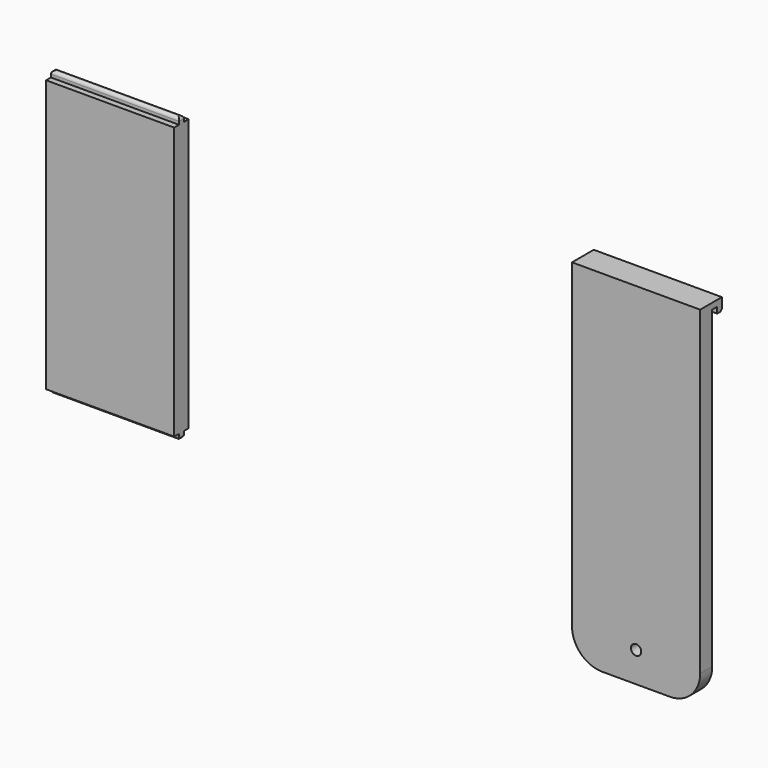
from build123d import *

# Parameters (mm, degrees)
F0_W      = 53.848
F0_H      = 114.3
F1_DEPTH  = 7.62
F2_W      = 2.54
F2_H      = 2.54
F3_DEPTH  = 53.848
F4_R      = 1.26999
F5_R      = 1.26999
F6_W      = 53.848
F6_H      = 147.32
F7_DEPTH  = 6.35
F8_R      = 12.7
F9_W      = 53.848
F9_H      = 5.08
F10_DEPTH = 5.08
F11_W     = 2.54
F11_H     = 2.54
F12_DEPTH = 76.2
F13_SIZE  = 0.762
F14_R     = 2.159
F15_DEPTH = 25.4


# Not quite as in the source:
# - a fillet or chamfer is up to 0.001 mm smaller than in the source, because OpenCascade refuses the exact size


with BuildPart() as f1:
    # F0 (on Front) → F1 (new body)
    with BuildSketch(Plane.XZ):
        with Locations((-110.2400206625, 2.555437386)):
            Rectangle(F0_W, F0_H)
    extrude(amount=F1_DEPTH)

    # F2 (on face) → F3 (join)
    with BuildSketch(Plane(origin=(-137.1640206625, 0, 0), x_dir=(0, -1, 0), z_dir=(-1, 0, 0))):
        with Locations((3.81, -55.864562614)):
            Rectangle(F2_W, F2_H)
        with Locations((3.81, 60.975437386)):
            Rectangle(F2_W, F2_H)
    extrude(amount=-F3_DEPTH)

    # F4 (radius 1.27 in the source; OpenCascade refuses exactly that, so slightly less here)
    f4_edges = [f1.edges().sort_by_distance(p)[0] for p in [
        (-110.240021, -2.54, 62.245437),
        (-110.240021, -5.08, 62.245437),
        (-137.164021, -3.81, 62.245437),
        (-83.316021, -3.81, 62.245437),
    ]]
    fillet(f4_edges, radius=F4_R)

    # F5 (radius 1.27 in the source; OpenCascade refuses exactly that, so slightly less here)
    f5_edges = [f1.edges().sort_by_distance(p)[0] for p in [
        (-110.240021, -5.08, -57.134563),
        (-110.240021, -2.54, -57.134563),
        (-83.316021, -3.81, -57.134563),
        (-137.164021, -3.81, -57.134563),
    ]]
    fillet(f5_edges, radius=F5_R)


with BuildPart() as f7:
    # F6 (on Front) → F7 (new body)
    with BuildSketch(Plane.XZ):
        with Locations((109.727306695, -10.2860404956)):
            Rectangle(F6_W, F6_H)
    extrude(amount=F7_DEPTH)

    # F8
    f8_edges = [f7.edges().sort_by_distance(p)[0] for p in [
        (136.651307, -3.175, -83.94604),
        (82.803307, -3.175, -83.94604),
    ]]
    fillet(f8_edges, radius=F8_R)

    # F9 (on face) → F10 (join)
    with BuildSketch(Plane(origin=(0, 0, 0), x_dir=(-1, 0, 0), z_dir=(0, 1, 0))):
        with Locations((-109.727306695, 60.8339595044)):
            Rectangle(F9_W, F9_H)
    extrude(amount=F10_DEPTH)

    # F11 (on face) → F12 (cut)
    with BuildSketch(Plane(origin=(82.803306695, 0, 0), x_dir=(0, -1, 0), z_dir=(-1, 0, 0))):
        with Locations((-1.27, 59.5639595044)):
            Rectangle(F11_W, F11_H)
    extrude(amount=-F12_DEPTH, mode=Mode.SUBTRACT)

    # F13
    f13_edges = [f7.edges().sort_by_distance(p)[0] for p in [
        (109.727307, 5.08, 58.29396),
    ]]
    chamfer(f13_edges, length=F13_SIZE)

    # F14 (on face) → F15 (cut)
    with BuildSketch(Plane(origin=(0, 0, 0), x_dir=(-1, 0, 0), z_dir=(0, 1, 0))):
        with Locations((-109.727306695, -71.2460404956)):
            Circle(F14_R)
    extrude(amount=-F15_DEPTH, mode=Mode.SUBTRACT)


solid = Compound([f1.part, f7.part])
